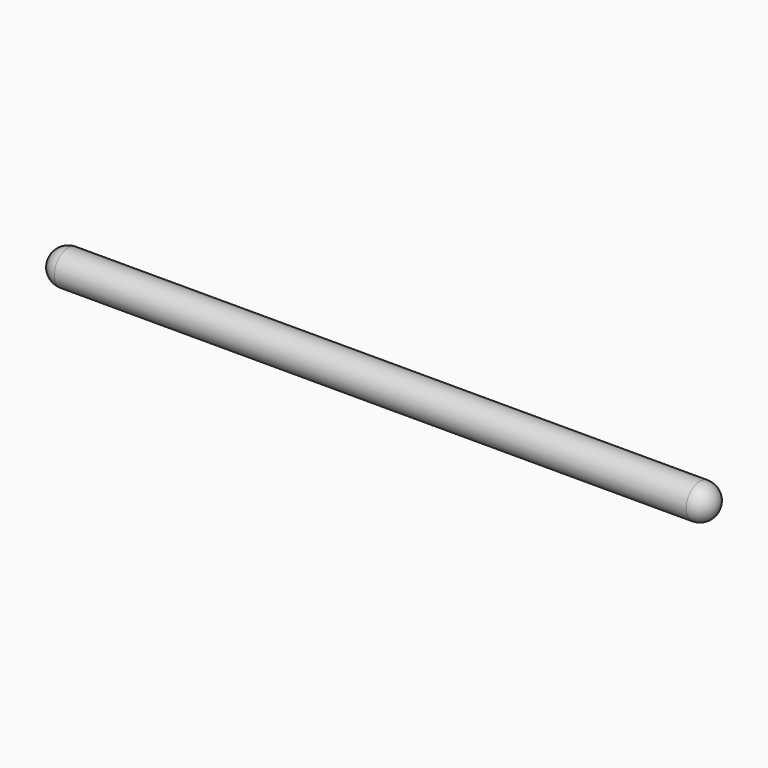
from build123d import *


# Not quite as in the source:
# - a feature names something its author has since deleted; it is built from what else it names


with BuildPart() as f1:
    # F0 (on Front) → F1 (revolve)
    with BuildSketch(Plane.XZ):
        with BuildLine():
            Line((92.2147, 0), (0, 0))
            ThreePointArc((0, 0), (1.3949039546, -3.3675960454), (4.7625, -4.7625))
            Line((4.7625, -4.7625), (179.6669, -4.7625))
            ThreePointArc((179.6669, -4.7625), (183.0344960454, -3.3675960454), (184.4294, 0))
            Line((184.4294, 0), (179.6669, 0))
            Line((179.6669, 0), (92.2147, 0))
        make_face()
    revolve(axis=Axis((46.10735, 0, 0), (-1, 0, 0)))


solid = f1.part
